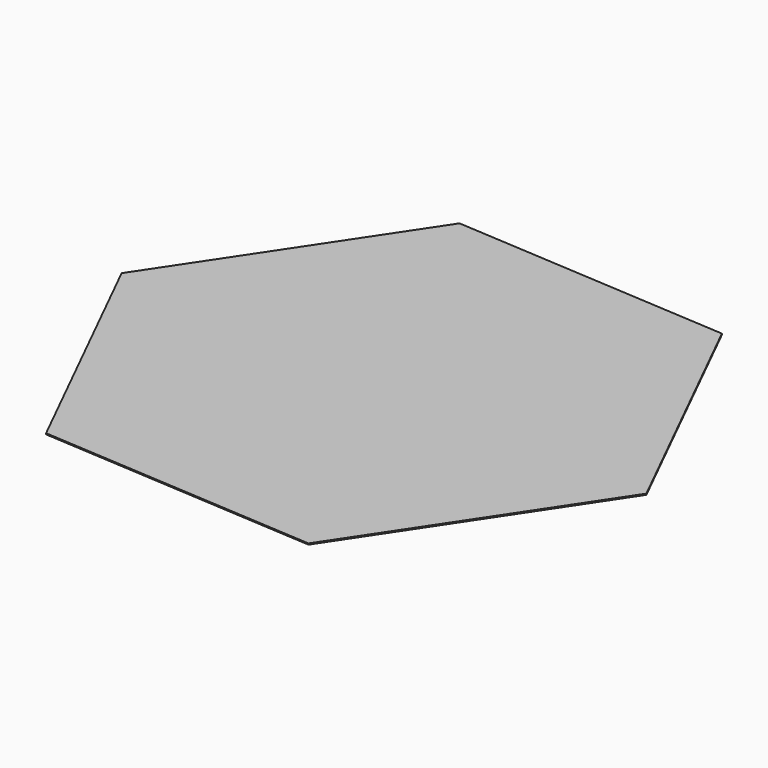
from build123d import *

# Parameters (mm, degrees)
F2_DEPTH = 0.1


with BuildPart() as f2:
    # F1 (on Top) → F2 (new body)
    with BuildSketch(Plane.XY):
        Polygon((24.9496552483, -1.5857815073), (13.8481546943, 20.8141445071), (-11.101500554, 22.3999260144), (-24.9496552483, 1.5857815073), (-13.8481546943, -20.8141445071), (11.101500554, -22.3999260144), align=None)
    extrude(amount=F2_DEPTH)


solid = f2.part
